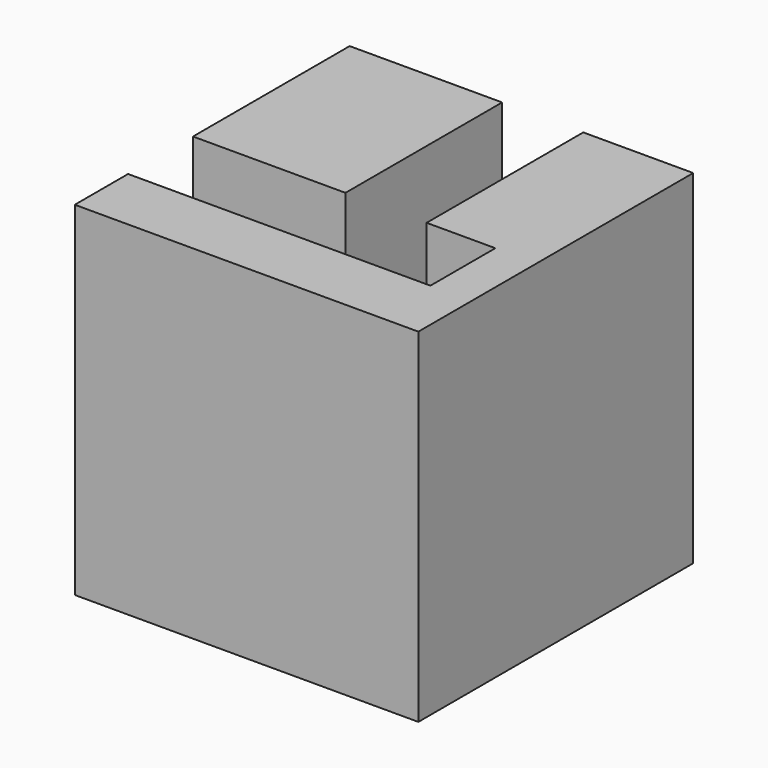
from build123d import *

# Parameters (mm, degrees)
F0_W     = 5.636
F0_H     = 7.2381474632
F1_DEPTH = 10.16
F2_W     = 5.636
F2_H     = 7.2381474632
F3_DEPTH = 2.54


# Not quite as in the source:
# - a feature of the source that left no trace in its solid (it failed there, or was rolled back) is left out


with BuildPart() as f1:
    # F0 (on Top) → F1 (new body)
    with BuildSketch(Plane.XY):
        with Locations((-5.0819813066, -2.7033329925)):
            Rectangle(F0_W, F0_H)
    extrude(amount=F1_DEPTH)



with BuildPart() as f1b:
    # F0 (on Top) → F1, piece 2 (new body)
    with BuildSketch(Plane.XY):
        Polygon((-10.8999813066, 0.9157407391), (-14.9639813066, 0.9157407391), (-14.9639813066, -11.7842592609), (-2.2639813066, -11.7842592609), (-2.2639813066, -9.3224067241), (-7.8999813066, -9.3224067241), (-10.8999813066, -9.3224067241), (-13.4399813066, -9.3224067241), (-13.4399813066, -6.3224067241), (-10.8999813066, -6.3224067241), align=None)
    extrude(amount=F1_DEPTH)


with BuildPart() as f1_1:
    add(f1.part)

    add(f1b.part)  # F3 merges F1b
    # F2 (on face) → F3 (join)
    with BuildSketch(Plane(origin=(0, 0, 0), x_dir=(1, 0, 0), z_dir=(0, 0, -1))):
        with Locations((-5.0819813066, 2.7033329925)):
            Rectangle(F2_W, F2_H)
        Polygon((-2.2639813066, 9.3224067241), (-13.4399813066, 9.3224067241), (-13.4399813066, 6.3224067241), (-10.8999813066, 6.3224067241), (-10.8999813066, -0.9157407391), (-7.8999813066, -0.9157407391), (-7.8999813066, 6.3224067241), (-2.2639813066, 6.3224067241), align=None)
        Polygon((-13.4399813066, 6.3224067241), (-13.4399813066, 9.3224067241), (-2.2639813066, 9.3224067241), (-2.2639813066, 11.7842592609), (-14.9639813066, 11.7842592609), (-14.9639813066, -0.9157407391), (-10.8999813066, -0.9157407391), (-10.8999813066, 6.3224067241), align=None)
    extrude(amount=F3_DEPTH)


with BuildPart() as f5_1:
    # F5: instance of F1
    add(f1_1.part.mirror(Plane(origin=(-8.6139813066, -4.877797716, 3.5140776699), x_dir=(0, 1, 0), z_dir=(1, 0, 0))))


solid = f5_1.part
